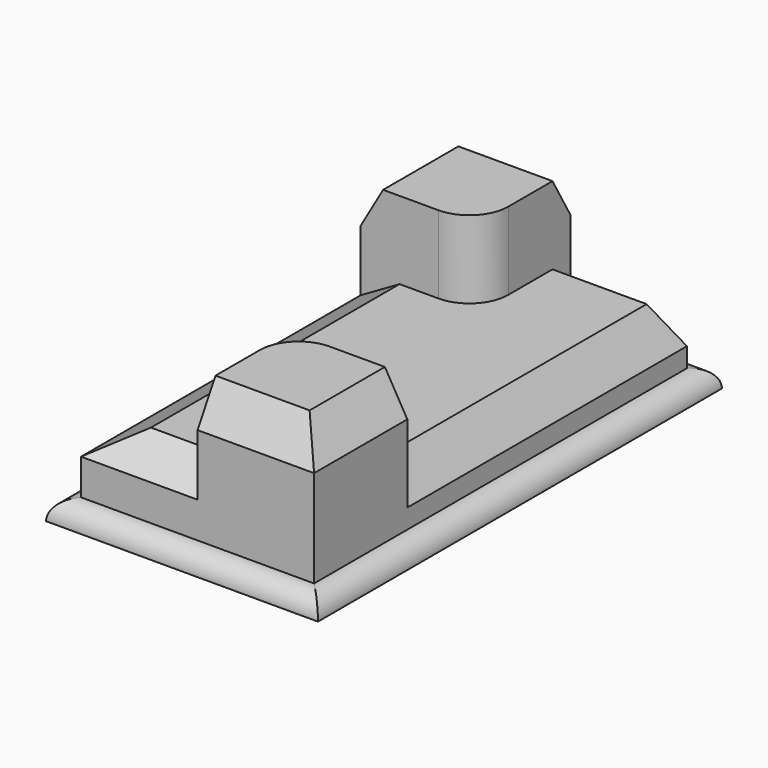
from build123d import *

# Parameters (mm, degrees)
F0_W        = 88.9
F0_H        = 165.1
F1_DEPTH    = 6.35
F2_DEPTH    = 25.4
F3_DEPTH    = 50.8
F4_R        = 6.34999
F5_C1_SIZE2 = 7.3323484187
F5_C1_SIZE  = 12.7
F5_C2_SIZE2 = 12.7
F5_C2_SIZE  = 7.3323484187
F5_C3_SIZE2 = 7.3323484187
F5_C3_SIZE  = 12.7
F5_C4_SIZE2 = 7.3323484187
F5_C4_SIZE  = 12.7
F5_C5_SIZE2 = 7.3323484187
F5_C5_SIZE  = 12.7
F5_C6_SIZE2 = 7.3323484187
F5_C6_SIZE  = 12.7
F6_C1_SIZE2 = 7.3323484187
F6_C1_SIZE  = 12.7
F6_C2_SIZE2 = 12.7
F6_C2_SIZE  = 7.3323484187


# Not quite as in the source:
# - a fillet or chamfer is up to 0.001 mm smaller than in the source, because OpenCascade refuses the exact size


with BuildPart() as f1:
    # F0 (on Top) → F1 (new body)
    with BuildSketch(Plane.XY):
        with Locations((-14.4346988976, -1.2875000358)):
            Rectangle(F0_W, F0_H)
        Polygon((-52.5346988976, 36.8124999642), (-52.5346988976, 74.9124999642), (-14.4346988976, 74.9124999642), (23.6653011024, 74.9124999642), (23.6653011024, -39.3875000358), (23.6653011024, -77.4875000358), (-14.4346988976, -77.4875000358), (-52.5346988976, -77.4875000358), align=None, mode=Mode.SUBTRACT)
    extrude(amount=F1_DEPTH)

    # F0 (on Top) → F2 (join)
    with BuildSketch(Plane.XY):
        with BuildLine():
            Line((23.6653011024, 74.9124999642), (-14.4346988976, 74.9124999642))
            Line((-14.4346988976, 74.9124999642), (-14.4346988976, 49.5124999642))
            ThreePointArc((-14.4346988976, 49.5124999642), (-18.1544427765, 40.5322438432), (-27.1346988976, 36.8124999642))
            Line((-27.1346988976, 36.8124999642), (-52.5346988976, 36.8124999642))
            Line((-52.5346988976, 36.8124999642), (-52.5346988976, -77.4875000358))
            Line((-52.5346988976, -77.4875000358), (-14.4346988976, -77.4875000358))
            Line((-14.4346988976, -77.4875000358), (-14.4346988976, -52.0875000358))
            ThreePointArc((-14.4346988976, -52.0875000358), (-10.7149550187, -43.1072439147), (-1.7346988976, -39.3875000358))
            Line((-1.7346988976, -39.3875000358), (23.6653011024, -39.3875000358))
            Line((23.6653011024, -39.3875000358), (23.6653011024, 74.9124999642))
        make_face()
    extrude(amount=F2_DEPTH)

    # F0 (on Top) → F3 (join)
    with BuildSketch(Plane.XY):
        with BuildLine():
            Line((-14.4346988976, 74.9124999642), (-52.5346988976, 74.9124999642))
            Line((-52.5346988976, 74.9124999642), (-52.5346988976, 36.8124999642))
            Line((-52.5346988976, 36.8124999642), (-27.1346988976, 36.8124999642))
            ThreePointArc((-27.1346988976, 36.8124999642), (-18.1544427765, 40.5322438432), (-14.4346988976, 49.5124999642))
            Line((-14.4346988976, 49.5124999642), (-14.4346988976, 74.9124999642))
        make_face()
        with BuildLine():
            Line((23.6653011024, -77.4875000358), (23.6653011024, -39.3875000358))
            Line((23.6653011024, -39.3875000358), (-1.7346988976, -39.3875000358))
            ThreePointArc((-1.7346988976, -39.3875000358), (-10.7149550187, -43.1072439147), (-14.4346988976, -52.0875000358))
            Line((-14.4346988976, -52.0875000358), (-14.4346988976, -77.4875000358))
            Line((-14.4346988976, -77.4875000358), (23.6653011024, -77.4875000358))
        make_face()
    extrude(amount=F3_DEPTH)

    # F4 (radius 6.35 in the source; OpenCascade refuses exactly that, so slightly less here)
    f4_edges = [f1.edges().sort_by_distance(p)[0] for p in [
        (-14.434699, -83.8375, 6.35),
        (-14.434699, 81.2625, 6.35),
        (30.015301, -1.2875, 6.35),
        (-58.884699, -1.2875, 6.35),
    ]]
    fillet(f4_edges, radius=F4_R)

    # F5: chamfer of 12.7 x 7.3323484187 on 6 edges, made by hand

    # F5_c1
    f5_c1_edges = [f1.edges().sort_by_distance(p)[0] for p in [
        (-52.5346988976, 55.8624999642, 50.8),
    ]]
    f5_c1_side = f1.faces().sort_by_distance((-52.5346988976, 55.8624999642, 50.6533530316))[0]
    chamfer(f5_c1_edges, length=F5_C1_SIZE, length2=F5_C1_SIZE2, reference=f5_c1_side)

    # F5_c2
    f5_c2_edges = [f1.edges().sort_by_distance(p)[0] for p in [
        (-52.5346988976, -20.3375000358, 25.4),
    ]]
    f5_c2_side = f1.faces().sort_by_distance((-52.5346988976, -20.3375000358, 25.2533530316))[0]
    chamfer(f5_c2_edges, length=F5_C2_SIZE, length2=F5_C2_SIZE2, reference=f5_c2_side)

    # F5_c3
    f5_c3_edges = [f1.edges().sort_by_distance(p)[0] for p in [
        (4.6153011024, 74.9124999642, 25.4),
    ]]
    f5_c3_side = f1.faces().sort_by_distance((4.6153011024, 74.9124999642, 25.2533530316))[0]
    chamfer(f5_c3_edges, length=F5_C3_SIZE, length2=F5_C3_SIZE2, reference=f5_c3_side)

    # F5_c4
    f5_c4_edges = [f1.edges().sort_by_distance(p)[0] for p in [
        (-29.8185246882, 74.9124999642, 50.8),
    ]]
    f5_c4_side = f1.faces().sort_by_distance((-29.8185246882, 74.9124999642, 50.6533530316))[0]
    chamfer(f5_c4_edges, length=F5_C4_SIZE, length2=F5_C4_SIZE2, reference=f5_c4_side)

    # F5_c5
    f5_c5_edges = [f1.edges().sort_by_distance(p)[0] for p in [
        (23.6653011024, 14.0963257549, 25.4),
    ]]
    f5_c5_side = f1.faces().sort_by_distance((23.6653011024, 14.0963257549, 25.2533530316))[0]
    chamfer(f5_c5_edges, length=F5_C5_SIZE, length2=F5_C5_SIZE2, reference=f5_c5_side)

    # F5_c6
    f5_c6_edges = [f1.edges().sort_by_distance(p)[0] for p in [
        (-27.1346988976, -77.4875000358, 25.4),
    ]]
    f5_c6_side = f1.faces().sort_by_distance((-27.1346988976, -77.3408530674, 25.4))[0]
    chamfer(f5_c6_edges, length=F5_C6_SIZE, length2=F5_C6_SIZE2, reference=f5_c6_side)

    # F6: chamfer of 12.7 x 7.3323484187 on 2 edges, made by hand

    # F6_c1
    f6_c1_edges = [f1.edges().sort_by_distance(p)[0] for p in [
        (4.6153011024, -77.4875000358, 50.8),
    ]]
    f6_c1_side = f1.faces().sort_by_distance((4.6153011024, -77.4875000358, 50.6533530316))[0]
    chamfer(f6_c1_edges, length=F6_C1_SIZE, length2=F6_C1_SIZE2, reference=f6_c1_side)

    # F6_c2
    f6_c2_edges = [f1.edges().sort_by_distance(p)[0] for p in [
        (23.6653011024, -54.7713258264, 50.8),
    ]]
    f6_c2_side = f1.faces().sort_by_distance((23.518654134, -54.7713258264, 50.8))[0]
    chamfer(f6_c2_edges, length=F6_C2_SIZE, length2=F6_C2_SIZE2, reference=f6_c2_side)


solid = f1.part
